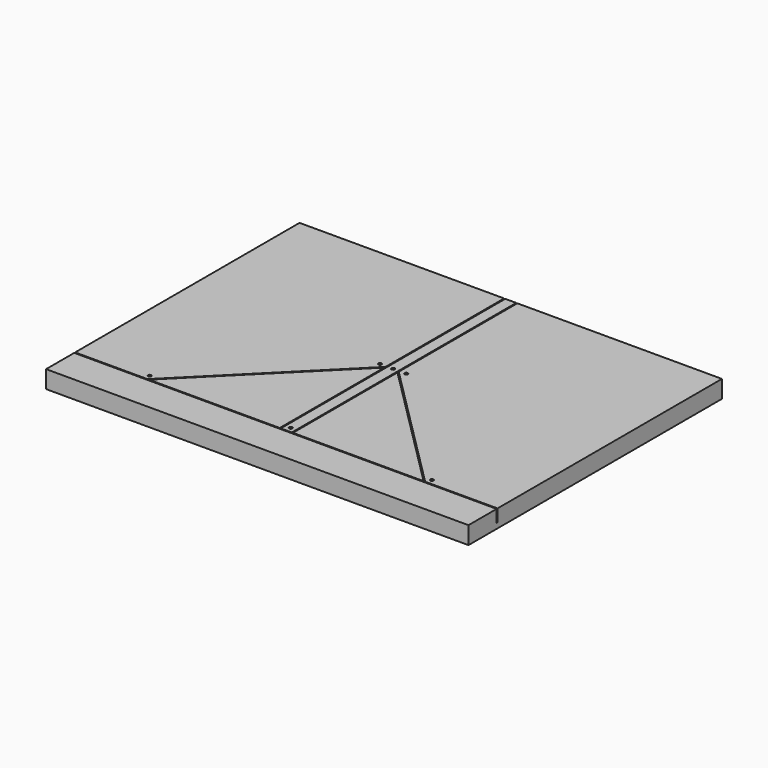
from build123d import *

# Parameters (mm, degrees)
F0_W     = 1219.2
F0_H     = 914.4
F1_DEPTH = 50.8
F2_W     = 3.175
F2_H     = 34.925
F3_DEPTH = 35.56
F4_R     = 4.7625
F5_DEPTH = 50.801


with BuildPart() as f1:
    # F0 (on Top) → F1 (new body)
    with BuildSketch(Plane.XY):
        with Locations((609.6, 457.2)):
            Rectangle(F0_W, F0_H)
    extrude(amount=F1_DEPTH)

    # F2 (on face) → F3 (cut)
    with BuildSketch(Plane.XY.offset(50.8)):
        Polygon((590.55, 486.4358851454), (243.8141148546, 139.7), (248.3042429151, 139.7), (590.55, 481.9457570849), align=None)
        Polygon((590.55, 914.4), (590.55, 535.8272938113), (590.55, 486.4358851454), (590.55, 481.9457570849), (590.55, 139.7), (593.725, 139.7), (593.725, 914.4), align=None)
        Polygon((970.8957570849, 139.7), (975.3858851454, 139.7), (628.65, 486.4358851454), (628.65, 481.9457570849), align=None)
        with Locations((592.1375, 122.2375)):
            Rectangle(F2_W, F2_H)
        Polygon((0, 104.775), (0, 101.6), (1219.2, 101.6), (1219.2, 104.775), (1059.7022938113, 104.775), (1010.3108851454, 104.775), (1005.8207570849, 104.775), (628.65, 104.775), (625.475, 104.775), (593.725, 104.775), (590.55, 104.775), (213.3792429151, 104.775), (208.8891148546, 104.775), (159.4977061887, 104.775), align=None)
        Polygon((243.8141148546, 139.7), (208.8891148546, 104.775), (213.3792429151, 104.775), (248.3042429151, 139.7), align=None)
        Polygon((1005.8207570849, 104.775), (1010.3108851454, 104.775), (975.3858851454, 139.7), (970.8957570849, 139.7), align=None)
        Polygon((628.65, 486.4358851454), (628.65, 535.8272938113), (628.65, 914.4), (625.475, 914.4), (625.475, 139.7), (628.65, 139.7), (628.65, 481.9457570849), align=None)
        with Locations((627.0625, 122.2375)):
            Rectangle(F2_W, F2_H)
    extrude(amount=-F3_DEPTH, mode=Mode.SUBTRACT)

    # F4 (on face) → F5 (cut, through all)
    with BuildSketch(Plane.XY.offset(50.8)):
        with Locations((202.3134745519, 120.65)):
            Circle(F4_R)
        with Locations((571.5, 489.8365254481)):
            Circle(F4_R)
        with Locations((609.6, 489.8365254481)):
            Circle(F4_R)
        with Locations((647.7, 489.8365254481)):
            Circle(F4_R)
        with Locations((609.6, 120.65)):
            Circle(F4_R)
        with Locations((1016.8865254481, 120.65)):
            Circle(F4_R)
    extrude(amount=-F5_DEPTH, mode=Mode.SUBTRACT)


solid = f1.part
